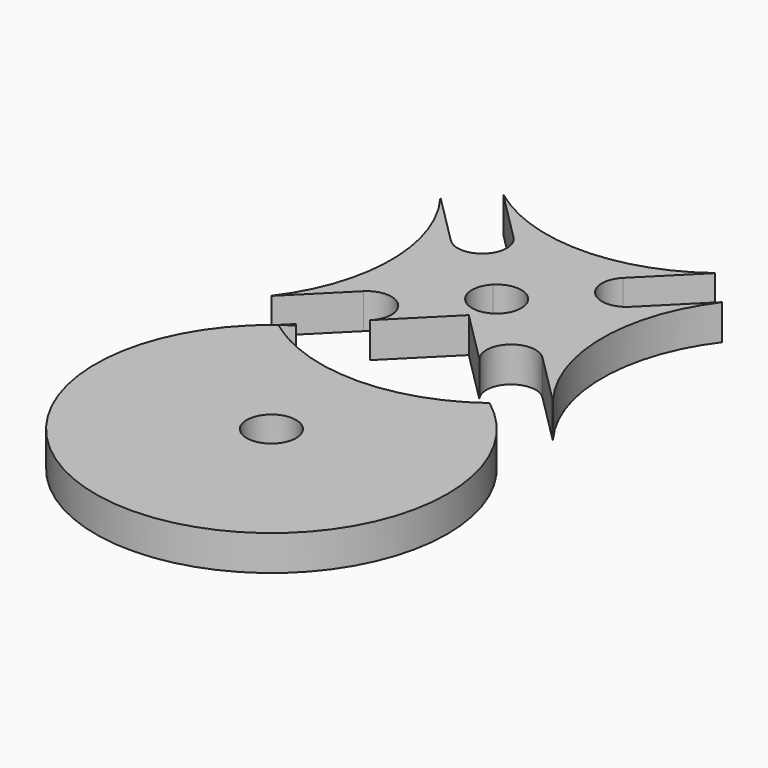
from build123d import *

# Parameters (mm, degrees)
F1_DEPTH = 5


# Not quite as in the source:
# - a feature names something its author has since deleted; it is built from what else it names


with BuildPart() as f1:
    # F0 (on Top) → F1 (new body)
    with BuildSketch(Plane.XY):
        with BuildLine():
            ThreePointArc((-9.9073162791, 17.0468938018), (-12.5408855394, 18.3730217116), (-15, 20))
            ThreePointArc((-15, 20), (-16.2829033321, 18.9701623366), (-17.4952976137, 17.8581791179))
            Line((-17.4952976137, 17.8581791179), (-2.8184302399, -2.0751990225))
            ThreePointArc((-2.8184302399, -2.0751990225), (-2.172900388, 2.7438119294), (2.6658084384, 2.2679209355))
            Line((2.6658084384, 2.2679209355), (-9.9073162791, 17.0468938018))
        make_face()
        with BuildLine():
            Line((-2.8184302399, -2.0751990225), (-17.4952976137, 17.8581791179))
            ThreePointArc((-17.4952976137, 17.8581791179), (1.6442252637, -24.9458718685), (15, 20))
            ThreePointArc((15, 20), (2.9434785416, 15.1738860456), (-9.9073162791, 17.0468938018))
            Line((-9.9073162791, 17.0468938018), (2.6658084384, 2.2679209355))
            ThreePointArc((2.6658084384, 2.2679209355), (3.2848386212, 1.2082364143), (3.5, 0))
            ThreePointArc((3.5, 0), (1.0921296078, -3.325244791), (-2.8184302399, -2.0751990225))
        make_face()
    extrude(amount=F1_DEPTH)


with BuildPart() as f1b:
    # F0 (on Top) → F1, piece 2 (new body)
    with BuildSketch(Plane.XY):
        with BuildLine():
            ThreePointArc((-15.0286973301, 20.0215552016), (-15.0143525332, 20.0107724509), (-15, 20))
            ThreePointArc((-15, 20), (-14.1981285052, 20.5770052959), (-13.3740867349, 21.1218797461))
            Line((-13.3740867349, 21.1218797461), (-13.6288791735, 21.4213733582))
            Line((-13.6288791735, 21.4213733582), (-15.0286973301, 20.0215552016))
        make_face()
    extrude(amount=F1_DEPTH)


with BuildPart() as f1c:
    # F0 (on Top) → F1, piece 3 (new body)
    with BuildSketch(Plane.XY):
        with BuildLine():
            ThreePointArc((-12.7279220614, 32.2218254069), (-7.7781745931, 32.2218254069), (-7.7781745931, 27.2720779386))
            Line((-7.7781745931, 27.2720779386), (0, 35.0502525317))
            Line((0, 35.0502525317), (-2.4748737374, 37.5251262691))
            Line((-2.4748737374, 37.5251262691), (-4.9497474683, 40))
            Line((-4.9497474683, 40), (-12.7279220614, 32.2218254069))
        make_face()
        with BuildLine():
            Line((0, 35.0502525317), (7.7781745931, 27.2720779386))
            ThreePointArc((7.7781745931, 27.2720779386), (7.7781745931, 32.2218254069), (12.7279220614, 32.2218254069))
            Line((12.7279220614, 32.2218254069), (4.9497474683, 40))
            Line((4.9497474683, 40), (2.4748737427, 37.5251262744))
            Line((2.4748737427, 37.5251262744), (0, 35.0502525317))
        make_face()
        with BuildLine():
            Line((12.7279220614, 32.2218254069), (19.9784447984, 24.9713026699))
            ThreePointArc((19.9784447984, 24.9713026699), (19.9892275491, 24.9856474668), (20, 25))
            ThreePointArc((20, 25), (15, 40), (20, 55))
            ThreePointArc((20, 55), (19.9892275491, 55.0143525332), (19.9784447984, 55.0286973301))
            Line((19.9784447984, 55.0286973301), (12.7279220614, 47.7781745931))
            Line((12.7279220614, 47.7781745931), (4.9497474683, 40))
            Line((4.9497474683, 40), (12.7279220614, 32.2218254069))
        make_face()
        with BuildLine():
            ThreePointArc((-20, 25), (-19.9892275491, 24.9856474668), (-19.9784447984, 24.9713026699))
            Line((-19.9784447984, 24.9713026699), (-12.7279220614, 32.2218254069))
            Line((-12.7279220614, 32.2218254069), (-4.9497474683, 40))
            Line((-4.9497474683, 40), (-12.7279220614, 47.7781745931))
            Line((-12.7279220614, 47.7781745931), (-19.9784447984, 55.0286973301))
            ThreePointArc((-19.9784447984, 55.0286973301), (-19.9892275491, 55.0143525332), (-20, 55))
            ThreePointArc((-20, 55), (-15, 40), (-20, 25))
        make_face()
        with BuildLine():
            Line((-2.4748737374, 37.5251262691), (0, 35.0502525317))
            Line((0, 35.0502525317), (2.4748737427, 37.5251262744))
            ThreePointArc((2.4748737427, 37.5251262744), (3.7e-09, 36.5), (-2.4748737374, 37.5251262691))
        make_face()
        with BuildLine():
            Line((-4.9497474683, 40), (-2.4748737374, 37.5251262691))
            ThreePointArc((-2.4748737374, 37.5251262691), (-3.5, 40.0000000023), (-2.4748737342, 42.4748737342))
            Line((-2.4748737342, 42.4748737342), (-4.9497474683, 40))
        make_face()
        with BuildLine():
            ThreePointArc((3.5, 40), (3.2335783661, 38.6606079923), (2.4748737427, 37.5251262744))
            Line((2.4748737427, 37.5251262744), (4.9497474683, 40))
            Line((4.9497474683, 40), (2.4748737094, 42.4748737589))
            ThreePointArc((2.4748737094, 42.4748737589), (3.2335783571, 41.3393920295), (3.5, 40))
        make_face()
        with BuildLine():
            Line((-12.7279220614, 47.7781745931), (-4.9497474683, 40))
            Line((-4.9497474683, 40), (-2.4748737342, 42.4748737342))
            Line((-2.4748737342, 42.4748737342), (0, 44.9497474683))
            Line((0, 44.9497474683), (-7.7781745931, 52.7279220614))
            ThreePointArc((-7.7781745931, 52.7279220614), (-7.7781745931, 47.7781745931), (-12.7279220614, 47.7781745931))
        make_face()
        with BuildLine():
            Line((2.4748737094, 42.4748737589), (4.9497474683, 40))
            Line((4.9497474683, 40), (12.7279220614, 47.7781745931))
            ThreePointArc((12.7279220614, 47.7781745931), (7.7781745931, 47.7781745931), (7.7781745931, 52.7279220614))
            Line((7.7781745931, 52.7279220614), (0, 44.9497474683))
            Line((0, 44.9497474683), (2.4748737094, 42.4748737589))
        make_face()
        with BuildLine():
            Line((0, 44.9497474683), (-2.4748737342, 42.4748737342))
            ThreePointArc((-2.4748737342, 42.4748737342), (-1.75e-08, 43.5), (2.4748737094, 42.4748737589))
            Line((2.4748737094, 42.4748737589), (0, 44.9497474683))
        make_face()
        with BuildLine():
            Line((-7.7781745931, 52.7279220614), (0, 44.9497474683))
            Line((0, 44.9497474683), (7.7781745931, 52.7279220614))
            Line((7.7781745931, 52.7279220614), (15.0286973301, 59.9784447984))
            ThreePointArc((15.0286973301, 59.9784447984), (15.0143525332, 59.9892275491), (15, 60))
            ThreePointArc((15, 60), (0, 55), (-15, 60))
            ThreePointArc((-15, 60), (-15.0143525332, 59.9892275491), (-15.0286973301, 59.9784447984))
            Line((-15.0286973301, 59.9784447984), (-7.7781745931, 52.7279220614))
        make_face()
    extrude(amount=F1_DEPTH)


solid = Compound([f1.part, f1b.part, f1c.part])
